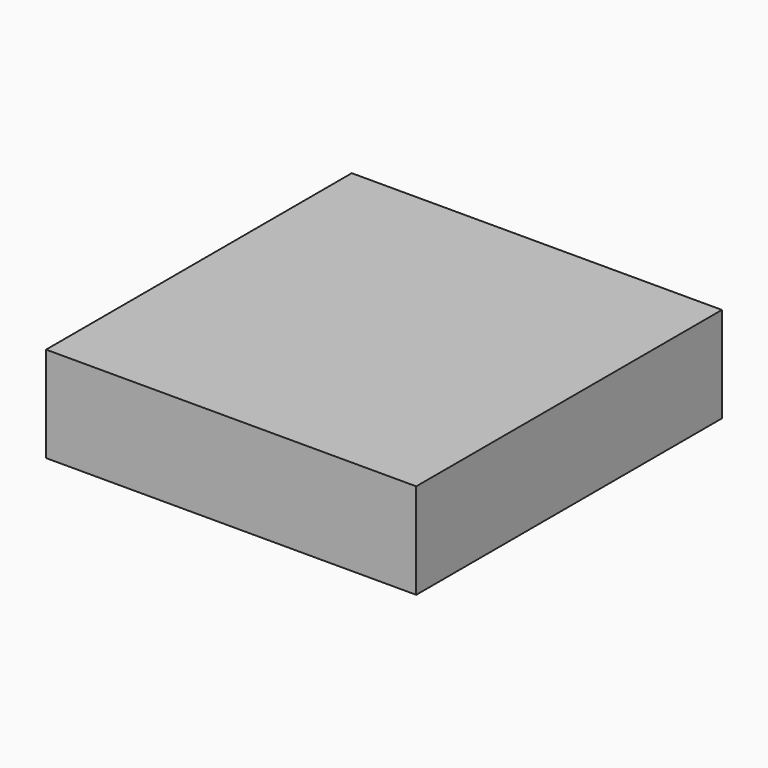
from build123d import *

# Parameters (mm, degrees)
F1_W     = 98.425
F1_H     = 101.6
F2_DEPTH = 25.4


# Not quite as in the source:
# - a variable given as a bare number and used for a length is read in inches; the dataset says mm whatever the document's units were


with BuildPart() as f2:
    # F1 (on Top) → F2 (new body)
    with BuildSketch(Plane.XY):
        Rectangle(F1_W, F1_H)
    extrude(amount=F2_DEPTH)


solid = f2.part
